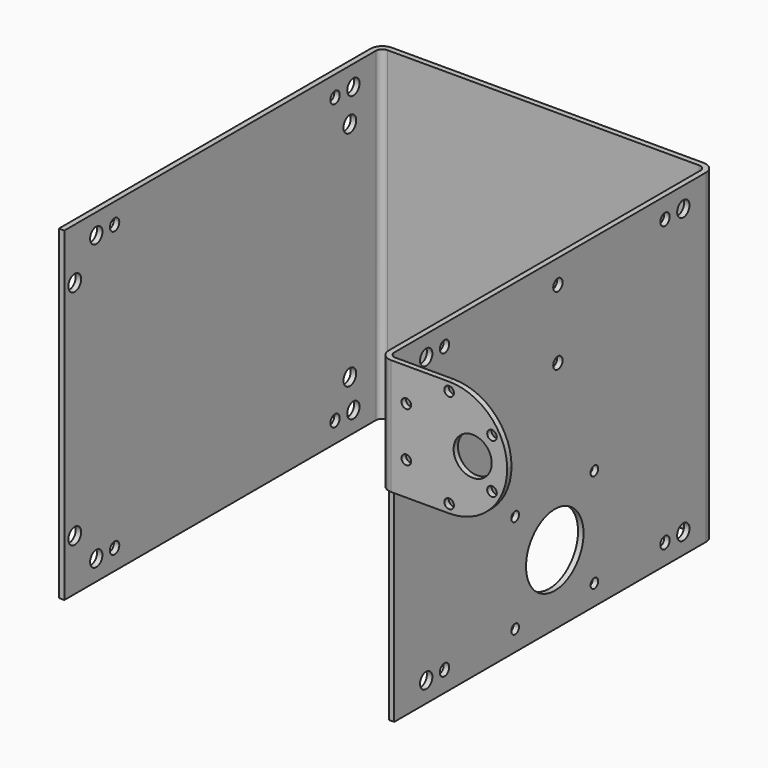
from build123d import *

# Parameters (mm, degrees)
F1_DEPTH  = 101.8535682
F2_R      = 1.5
F2_R_2    = 5.969
F3_DEPTH  = 1.70942
F4_R      = 1.98374
F5_R      = 3.69316
F6_R      = 2.4125047
F6_R_2    = 1.8288
F7_DEPTH  = 105.01884
F8_R      = 11.2530001
F8_R_2    = 1.5
F8_R_3    = 1.8288
F9_DEPTH  = 103.30942
F10_W     = 3.69316
F10_H     = 65.5315682
F11_DEPTH = 40.01516
F12_R     = 18.16099
F13_R     = 2.5
F14_DEPTH = 1.70942


# Not quite as in the source:
# - a fillet or chamfer is up to 0.001 mm smaller than in the source, because OpenCascade refuses the exact size
# - a feature names something its author has since deleted; it is built from what else it names


with BuildPart() as f1:
    # F0 (on Top) → F1 (new body)
    with BuildSketch(Plane.XY):
        Polygon((-1.70942, 0), (0, 0), (0, 123.945777), (101.6, 123.945777), (101.6, -3.69316), (141.61516, -3.69316), (141.61516, -1.98374), (103.30942, -1.98374), (103.30942, 125.655197), (-1.70942, 125.655197), align=None)
    extrude(amount=F1_DEPTH)

    # F2 (on face) → F3 (cut, through all)
    with BuildSketch(Plane.XZ.offset(3.69316)):
        with Locations((136.8723576062, 91.4395682)):
            Circle(F2_R)
        with Locations((130.82016, 83.6925682)):
            Circle(F2_R_2)
        with Locations((136.8723576062, 75.9455682)):
            Circle(F2_R)
        with Locations((123.45416, 99.1865682)):
            Circle(F2_R)
        with Locations((110.0359623938, 91.4395682)):
            Circle(F2_R)
        with Locations((110.0359623938, 75.9455682)):
            Circle(F2_R)
        with Locations((123.45416, 68.1985682)):
            Circle(F2_R)
    extrude(amount=-F3_DEPTH, mode=Mode.SUBTRACT)

    # F4
    f4_edges = [f1.edges().sort_by_distance(p)[0] for p in [
        (0, 123.945777, 50.926784),
        (101.6, 123.945777, 50.926784),
        (103.30942, -1.98374, 50.926784),
    ]]
    fillet(f4_edges, radius=F4_R)

    # F5
    f5_edges = [f1.edges().sort_by_distance(p)[0] for p in [
        (-1.70942, 125.655197, 50.926784),
        (103.30942, 125.655197, 50.926784),
        (101.6, -3.69316, 50.926784),
    ]]
    fillet(f5_edges, radius=F5_R)

    # F6 (on face) → F7 (cut, through all)
    with BuildSketch(Plane(origin=(-1.70942, 0, 0), x_dir=(0, -1, 0), z_dir=(-1, 0, 0))):
        with Locations((-12.5063584, 95.4723182)):
            Circle(F6_R)
        with Locations((-19.6813584, 95.4723182)):
            Circle(F6_R_2)
        with Locations((-105.9738466, 95.4723182)):
            Circle(F6_R_2)
        with Locations((-105.9738466, 6.38125)):
            Circle(F6_R_2)
        with Locations((-19.6813584, 6.38125)):
            Circle(F6_R_2)
        with Locations((-113.1488466, 95.4723182)):
            Circle(F6_R)
        with Locations((-113.1488466, 6.38125)):
            Circle(F6_R)
        with Locations((-12.5063584, 6.38125)):
            Circle(F6_R)
    extrude(amount=-F7_DEPTH, mode=Mode.SUBTRACT)

    # F8 (on face) → F9 (cut, through all)
    with BuildSketch(Plane.YZ.offset(103.30942)):
        with Locations((62.8276025004, 21.8812444)):
            Circle(F8_R)
        with Locations((47.3276081004, 37.3812388)):
            Circle(F8_R_2)
        with Locations((78.3275969004, 37.3812388)):
            Circle(F8_R_2)
        with Locations((78.3275969004, 6.38125)):
            Circle(F8_R_2)
        with Locations((47.3276081004, 6.38125)):
            Circle(F8_R_2)
        with Locations((64.05626, 72.9453964)):
            Circle(F8_R_3)
        with Locations((64.05626, 94.43974)):
            Circle(F8_R_3)
    extrude(amount=-F9_DEPTH, mode=Mode.SUBTRACT)

    # F10 (on face) → F11 (cut, through all)
    with BuildSketch(Plane.YZ.offset(141.61516)):
        with Locations((-1.84658, 32.7657841)):
            Rectangle(F10_W, F10_H)
    extrude(amount=-F11_DEPTH, mode=Mode.SUBTRACT)

    # F12 (radius 18.161 in the source; OpenCascade refuses exactly that, so slightly less here)
    f12_edges = [f1.edges().sort_by_distance(p)[0] for p in [
        (141.61516, -2.83845, 65.531568),
        (141.61516, -2.83845, 101.853568),
    ]]
    fillet(f12_edges, radius=F12_R)

    # F13 (on face) → F14 (cut, through all)
    with BuildSketch(Plane(origin=(-1.70942, 0, 0), x_dir=(0, -1, 0), z_dir=(-1, 0, 0))):
        with Locations((-111.7494286, 16.056229)):
            Circle(F13_R)
        with Locations((-4.0875, 16.056229)):
            Circle(F13_R)
        with Locations((-4.0875, 85.7973392)):
            Circle(F13_R)
        with Locations((-111.7494286, 85.7973392)):
            Circle(F13_R)
    extrude(amount=-F14_DEPTH, mode=Mode.SUBTRACT)


solid = f1.part
